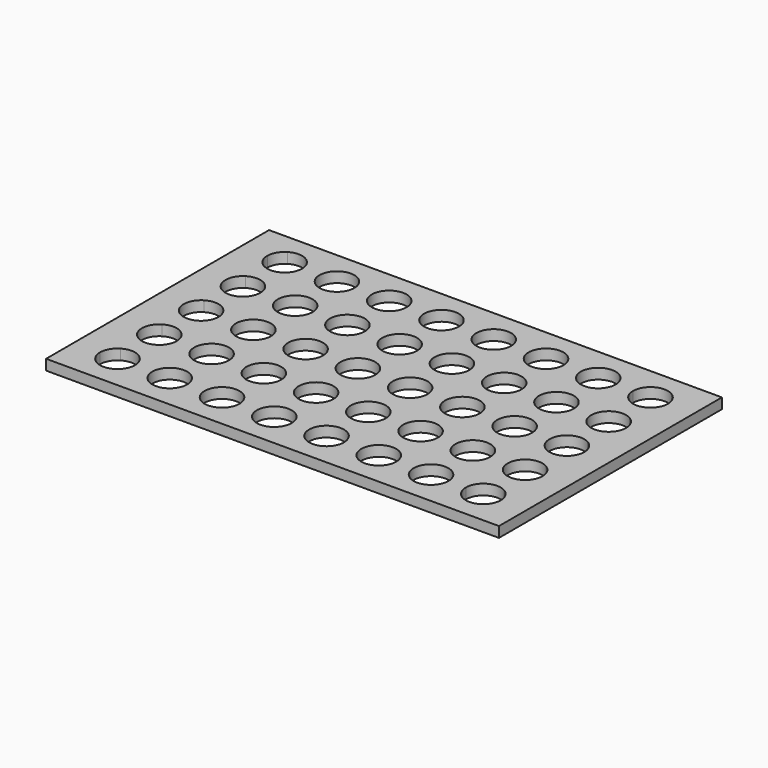
from build123d import *

# Parameters (mm, degrees)
F0_R     = 5
F1_DEPTH = 3


# Not quite as in the source:
# - a feature names something its author has since deleted; it is built from what else it names


with BuildPart() as f1:
    # F0 (on Top) → F1 (new body)
    with BuildSketch(Plane.XY):
        with BuildLine():
            Line((65, 30), (65, 40))
            Line((65, 40), (55, 40))
            Line((55, 40), (55, 34.3301270189))
            ThreePointArc((55, 34.3301270189), (56.8301270189, 32.5), (57.5, 30))
            Line((57.5, 30), (65, 30))
        make_face()
        with BuildLine():
            Line((55, 34.3301270189), (55, 40))
            Line((55, 40), (-55.1096590387, 40))
            Line((-55.1096590387, 40), (-55.1096590387, 34.2649360724))
            ThreePointArc((-55.1096590387, 34.2649360724), (-50.0554443342, 34.3616679833), (-47.5, 30))
            Line((-47.5, 30), (-42.5, 30))
            ThreePointArc((-42.5, 30), (-37.5, 35), (-32.5, 30))
            Line((-32.5, 30), (-27.5, 30))
            ThreePointArc((-27.5, 30), (-22.5, 35), (-17.5, 30))
            Line((-17.5, 30), (-12.5, 30))
            ThreePointArc((-12.5, 30), (-7.5, 35), (-2.5, 30))
            Line((-2.5, 30), (2.5, 30))
            ThreePointArc((2.5, 30), (7.5, 35), (12.5, 30))
            Line((12.5, 30), (17.5, 30))
            ThreePointArc((17.5, 30), (22.5, 35), (27.5, 30))
            Line((27.5, 30), (32.5, 30))
            ThreePointArc((32.5, 30), (37.5, 35), (42.5, 30))
            Line((42.5, 30), (47.5, 30))
            ThreePointArc((47.5, 30), (50, 34.3301270189), (55, 34.3301270189))
        make_face()
        with BuildLine():
            Line((65, -30), (65, 30))
            Line((65, 30), (57.5, 30))
            ThreePointArc((57.5, 30), (56.8301270189, 27.5), (55, 25.6698729811))
            Line((55, 25.6698729811), (55, 19.3301270189))
            ThreePointArc((55, 19.3301270189), (56.8301270189, 17.5), (57.5, 15))
            ThreePointArc((57.5, 15), (56.8301270189, 12.5), (55, 10.6698729811))
            Line((55, 10.6698729811), (55, 4.3301270189))
            ThreePointArc((55, 4.3301270189), (56.8301270189, 2.5), (57.5, 0))
            ThreePointArc((57.5, 0), (56.8301270189, -2.5), (55, -4.3301270189))
            Line((55, -4.3301270189), (55, -10.6698729811))
            ThreePointArc((55, -10.6698729811), (56.8301270189, -12.5), (57.5, -15))
            ThreePointArc((57.5, -15), (56.8301270189, -17.5), (55, -19.3301270189))
            Line((55, -19.3301270189), (55, -25.6698729811))
            ThreePointArc((55, -25.6698729811), (56.8301270189, -27.5), (57.5, -30))
            Line((57.5, -30), (65, -30))
        make_face()
        with BuildLine():
            Line((-55.1096590387, 34.2649360724), (-55.1096590387, 40))
            Line((-55.1096590387, 40), (-65, 40))
            Line((-65, 40), (-65, 30))
            Line((-65, 30), (-57.5, 30))
            ThreePointArc((-57.5, 30), (-56.8616679833, 32.4445556658), (-55.1096590387, 34.2649360724))
        make_face()
        with BuildLine():
            Line((65, -40), (65, -30))
            Line((65, -30), (57.5, -30))
            ThreePointArc((57.5, -30), (56.8301270189, -32.5), (55, -34.3301270189))
            Line((55, -34.3301270189), (55, -40))
            Line((55, -40), (65, -40))
        make_face()
        with BuildLine():
            ThreePointArc((55, 25.6698729811), (50, 25.6698729811), (47.5, 30))
            Line((47.5, 30), (42.5, 30))
            ThreePointArc((42.5, 30), (37.5, 25), (32.5, 30))
            Line((32.5, 30), (27.5, 30))
            ThreePointArc((27.5, 30), (22.5, 25), (17.5, 30))
            Line((17.5, 30), (12.5, 30))
            ThreePointArc((12.5, 30), (7.5, 25), (2.5, 30))
            Line((2.5, 30), (-2.5, 30))
            ThreePointArc((-2.5, 30), (-7.5, 25), (-12.5, 30))
            Line((-12.5, 30), (-17.5, 30))
            ThreePointArc((-17.5, 30), (-22.5, 25), (-27.5, 30))
            Line((-27.5, 30), (-32.5, 30))
            ThreePointArc((-32.5, 30), (-37.5, 25), (-42.5, 30))
            Line((-42.5, 30), (-47.5, 30))
            ThreePointArc((-47.5, 30), (-50.0554443342, 25.6383320167), (-55.1096590387, 25.7350639276))
            Line((-55.1096590387, 25.7350639276), (-55.1096590387, 19.2649360724))
            ThreePointArc((-55.1096590387, 19.2649360724), (-50.0554443342, 19.3616679833), (-47.5, 15))
            ThreePointArc((-47.5, 15), (-50.0554443342, 10.6383320167), (-55.1096590387, 10.7350639276))
            Line((-55.1096590387, 10.7350639276), (-55.1096590387, 4.2649360724))
            ThreePointArc((-55.1096590387, 4.2649360724), (-50.0554443342, 4.3616679833), (-47.5, 0))
            ThreePointArc((-47.5, 0), (-50.0554443342, -4.3616679833), (-55.1096590387, -4.2649360724))
            Line((-55.1096590387, -4.2649360724), (-55.1096590387, -10.7350639276))
            ThreePointArc((-55.1096590387, -10.7350639276), (-50.0554443342, -10.6383320167), (-47.5, -15))
            ThreePointArc((-47.5, -15), (-50.0554443342, -19.3616679833), (-55.1096590387, -19.2649360724))
            Line((-55.1096590387, -19.2649360724), (-55.1096590387, -25.7350639276))
            ThreePointArc((-55.1096590387, -25.7350639276), (-50.0554443342, -25.6383320167), (-47.5, -30))
            Line((-47.5, -30), (-42.5, -30))
            ThreePointArc((-42.5, -30), (-37.5, -25), (-32.5, -30))
            Line((-32.5, -30), (-27.5, -30))
            ThreePointArc((-27.5, -30), (-22.5, -25), (-17.5, -30))
            Line((-17.5, -30), (-12.5, -30))
            ThreePointArc((-12.5, -30), (-7.5, -25), (-2.5, -30))
            Line((-2.5, -30), (2.5, -30))
            ThreePointArc((2.5, -30), (7.5, -25), (12.5, -30))
            Line((12.5, -30), (17.5, -30))
            ThreePointArc((17.5, -30), (22.5, -25), (27.5, -30))
            Line((27.5, -30), (32.5, -30))
            ThreePointArc((32.5, -30), (37.5, -25), (42.5, -30))
            Line((42.5, -30), (47.5, -30))
            ThreePointArc((47.5, -30), (50, -25.6698729811), (55, -25.6698729811))
            Line((55, -25.6698729811), (55, -19.3301270189))
            ThreePointArc((55, -19.3301270189), (47.5, -15), (55, -10.6698729811))
            Line((55, -10.6698729811), (55, -4.3301270189))
            ThreePointArc((55, -4.3301270189), (47.5, 0), (55, 4.3301270189))
            Line((55, 4.3301270189), (55, 10.6698729811))
            ThreePointArc((55, 10.6698729811), (47.5, 15), (55, 19.3301270189))
            Line((55, 19.3301270189), (55, 25.6698729811))
        make_face()
        with Locations((-37.5, -15)):
            Circle(F0_R, mode=Mode.SUBTRACT)
        with Locations((-22.5, -15)):
            Circle(F0_R, mode=Mode.SUBTRACT)
        with Locations((-7.5, -15)):
            Circle(F0_R, mode=Mode.SUBTRACT)
        with Locations((-37.5, 0)):
            Circle(F0_R, mode=Mode.SUBTRACT)
        with Locations((-22.5, 0)):
            Circle(F0_R, mode=Mode.SUBTRACT)
        with Locations((-7.5, 0)):
            Circle(F0_R, mode=Mode.SUBTRACT)
        with Locations((7.5, -15)):
            Circle(F0_R, mode=Mode.SUBTRACT)
        with Locations((22.5, -15)):
            Circle(F0_R, mode=Mode.SUBTRACT)
        with Locations((7.5, 0)):
            Circle(F0_R, mode=Mode.SUBTRACT)
        with Locations((22.5, 0)):
            Circle(F0_R, mode=Mode.SUBTRACT)
        with Locations((37.5, -15)):
            Circle(F0_R, mode=Mode.SUBTRACT)
        with Locations((37.5, 0)):
            Circle(F0_R, mode=Mode.SUBTRACT)
        with Locations((-37.5, 15)):
            Circle(F0_R, mode=Mode.SUBTRACT)
        with Locations((-22.5, 15)):
            Circle(F0_R, mode=Mode.SUBTRACT)
        with Locations((-7.5, 15)):
            Circle(F0_R, mode=Mode.SUBTRACT)
        with Locations((7.5, 15)):
            Circle(F0_R, mode=Mode.SUBTRACT)
        with Locations((22.5, 15)):
            Circle(F0_R, mode=Mode.SUBTRACT)
        with Locations((37.5, 15)):
            Circle(F0_R, mode=Mode.SUBTRACT)
        with BuildLine():
            Line((-57.5, 30), (-65, 30))
            Line((-65, 30), (-65, -30))
            Line((-65, -30), (-57.5, -30))
            ThreePointArc((-57.5, -30), (-56.8616679833, -27.5554443342), (-55.1096590387, -25.7350639276))
            Line((-55.1096590387, -25.7350639276), (-55.1096590387, -19.2649360724))
            ThreePointArc((-55.1096590387, -19.2649360724), (-57.5, -15), (-55.1096590387, -10.7350639276))
            Line((-55.1096590387, -10.7350639276), (-55.1096590387, -4.2649360724))
            ThreePointArc((-55.1096590387, -4.2649360724), (-57.5, 0), (-55.1096590387, 4.2649360724))
            Line((-55.1096590387, 4.2649360724), (-55.1096590387, 10.7350639276))
            ThreePointArc((-55.1096590387, 10.7350639276), (-57.5, 15), (-55.1096590387, 19.2649360724))
            Line((-55.1096590387, 19.2649360724), (-55.1096590387, 25.7350639276))
            ThreePointArc((-55.1096590387, 25.7350639276), (-56.8616679833, 27.5554443342), (-57.5, 30))
        make_face()
        with BuildLine():
            Line((-55.1096590387, -40), (55, -40))
            Line((55, -40), (55, -34.3301270189))
            ThreePointArc((55, -34.3301270189), (50, -34.3301270189), (47.5, -30))
            Line((47.5, -30), (42.5, -30))
            ThreePointArc((42.5, -30), (37.5, -35), (32.5, -30))
            Line((32.5, -30), (27.5, -30))
            ThreePointArc((27.5, -30), (22.5, -35), (17.5, -30))
            Line((17.5, -30), (12.5, -30))
            ThreePointArc((12.5, -30), (7.5, -35), (2.5, -30))
            Line((2.5, -30), (-2.5, -30))
            ThreePointArc((-2.5, -30), (-7.5, -35), (-12.5, -30))
            Line((-12.5, -30), (-17.5, -30))
            ThreePointArc((-17.5, -30), (-22.5, -35), (-27.5, -30))
            Line((-27.5, -30), (-32.5, -30))
            ThreePointArc((-32.5, -30), (-37.5, -35), (-42.5, -30))
            Line((-42.5, -30), (-47.5, -30))
            ThreePointArc((-47.5, -30), (-50.0554443342, -34.3616679833), (-55.1096590387, -34.2649360724))
            Line((-55.1096590387, -34.2649360724), (-55.1096590387, -40))
        make_face()
        with BuildLine():
            Line((-57.5, -30), (-65, -30))
            Line((-65, -30), (-65, -40))
            Line((-65, -40), (-55.1096590387, -40))
            Line((-55.1096590387, -40), (-55.1096590387, -34.2649360724))
            ThreePointArc((-55.1096590387, -34.2649360724), (-56.8616679833, -32.4445556658), (-57.5, -30))
        make_face()
    extrude(amount=F1_DEPTH)


solid = f1.part
